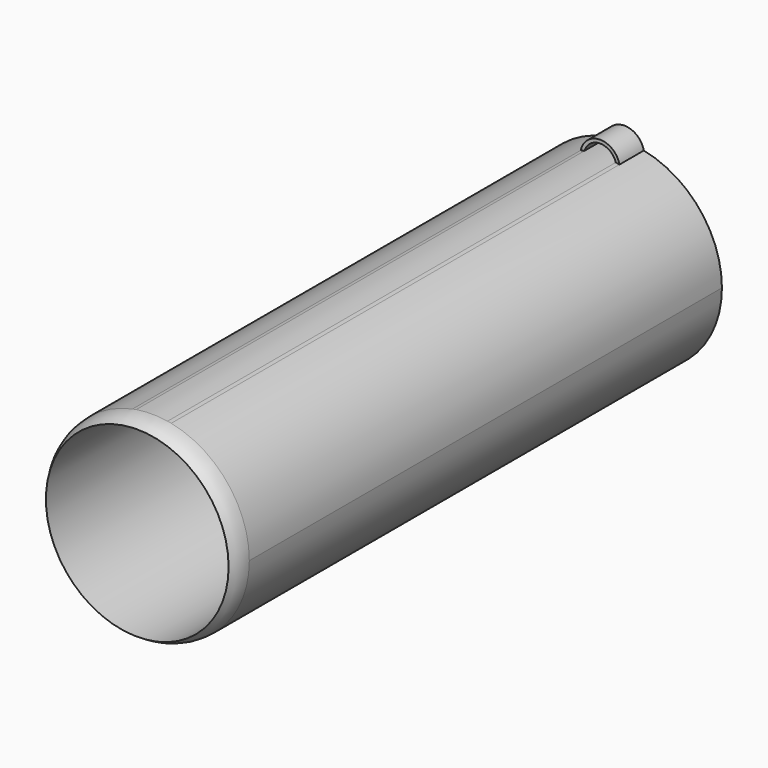
from build123d import *

# Parameters (mm, degrees)
F0_R     = 15
F1_DEPTH = 100
F2_DEPTH = 5


# Not quite as in the source:
# - a fillet or chamfer that OpenCascade refuses, or shapes differently, is made with other operations: its cross-section is extruded or revolved along the edge and cut away or added


with BuildPart() as f1:
    # F0 (on Front) → F1 (new body)
    with BuildSketch(Plane.XZ):
        with BuildLine():
            ThreePointArc((3.1768111268, 15.6814499031), (2.876945892, 15.7392243244), (2.5760326281, 15.7912651773))
            ThreePointArc((2.5760326281, 15.7912651773), (0, 16), (-2.5760326281, 15.7912651773))
            ThreePointArc((-2.5760326281, 15.7912651773), (-2.876945892, 15.7392243244), (-3.1768111268, 15.6814499031))
            ThreePointArc((-3.1768111268, 15.6814499031), (-10.1284505718, -12.3860602701), (16, 0))
            ThreePointArc((16, 0), (12.3860602701, 10.1284505718), (3.1768111268, 15.6814499031))
        make_face()
        Circle(F0_R, mode=Mode.SUBTRACT)
    extrude(amount=F1_DEPTH)

    # F0 (on Front) → F2 (join)
    with BuildSketch(Plane.XZ):
        with BuildLine():
            ThreePointArc((-2.5760326281, 15.7912651773), (0, 17.6948181166), (2.5760326281, 15.7912651773))
            ThreePointArc((2.5760326281, 15.7912651773), (2.876945892, 15.7392243244), (3.1768111268, 15.6814499031))
            ThreePointArc((3.1768111268, 15.6814499031), (0, 18.2490772391), (-3.1768111268, 15.6814499031))
            ThreePointArc((-3.1768111268, 15.6814499031), (-2.876945892, 15.7392243244), (-2.5760326281, 15.7912651773))
        make_face()
        with BuildLine():
            ThreePointArc((3.1768111268, 15.6814499031), (2.876945892, 15.7392243244), (2.5760326281, 15.7912651773))
            ThreePointArc((2.5760326281, 15.7912651773), (0, 16), (-2.5760326281, 15.7912651773))
            ThreePointArc((-2.5760326281, 15.7912651773), (-2.876945892, 15.7392243244), (-3.1768111268, 15.6814499031))
            ThreePointArc((-3.1768111268, 15.6814499031), (-10.1284505718, -12.3860602701), (16, 0))
            ThreePointArc((16, 0), (12.3860602701, 10.1284505718), (3.1768111268, 15.6814499031))
        make_face()
        Circle(F0_R, mode=Mode.SUBTRACT)
    extrude(amount=F2_DEPTH)

    # F3: fillet of radius 5 on 1 edges, made by hand

    # F3_s1 → F3_t2 (revolve, cut)
    with BuildSketch(Plane.XY):
        with BuildLine():
            ThreePointArc((16, -97), (15.7434164903, -98.5811388301), (15, -100))
            Line((15, -100), (16, -100))
            Line((16, -100), (16, -97))
        make_face()
    revolve(axis=Axis((0, -100, 0), (0, 1, 0)), mode=Mode.SUBTRACT)


solid = f1.part
